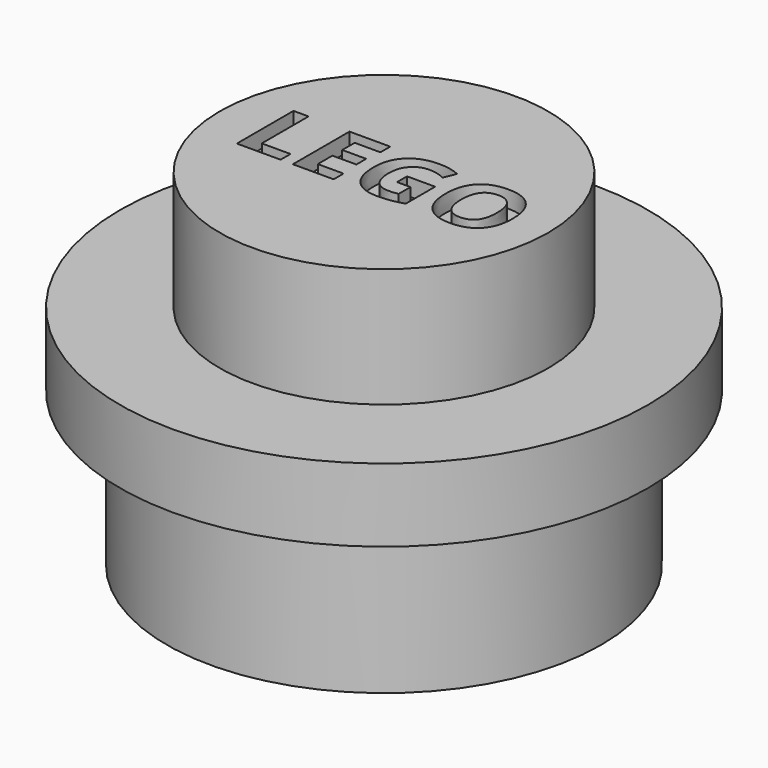
from build123d import *

# Parameters (mm, degrees)
F0_R         = 3.2385
F1_DEPTH     = 2.286
F2_R         = 3.937
F3_DEPTH     = 1.0922
F4_R         = 2.4511
F5_DEPTH     = 1.778
F6_T         = -0.762
F7_TEXT_SIZE = 1.4786040184
F8_DEPTH     = 0.254


# Not quite as in the source:
# - Text() gives the source's letters only with a copy of the font that has no kerning and outlines rounded to 1/6400 em; it was checked with that copy


with BuildPart() as f1:
    # F0 (on Top) → F1 (new body)
    with BuildSketch(Plane.XY):
        Circle(F0_R)
    extrude(amount=F1_DEPTH)

    # F2 (on face) → F3 (join)
    with BuildSketch(Plane.XY.offset(2.286)):
        Circle(F2_R)
    extrude(amount=F3_DEPTH)

    # F4 (on face) → F5 (join)
    with BuildSketch(Plane.XY.offset(3.3782)):
        Circle(F4_R)
    extrude(amount=F5_DEPTH)

    # F6
    f6_openings = [f1.faces().sort_by_distance(p)[0] for p in [
        (0, 0, 0),
    ]]
    offset(amount=F6_T, openings=f6_openings, kind=Kind.INTERSECTION)

    # F7 (on face) → F8 (cut)
    with BuildSketch(Plane.XY.offset(5.1562)):
        with Locations((-1.9196834182, -0.5096709356)):
            Text('LEGO', F7_TEXT_SIZE, font='Open Sans', font_style=FontStyle.BOLD, text_align=(TextAlign.LEFT, TextAlign.BOTTOM))
    extrude(amount=-F8_DEPTH, mode=Mode.SUBTRACT)


solid = f1.part
